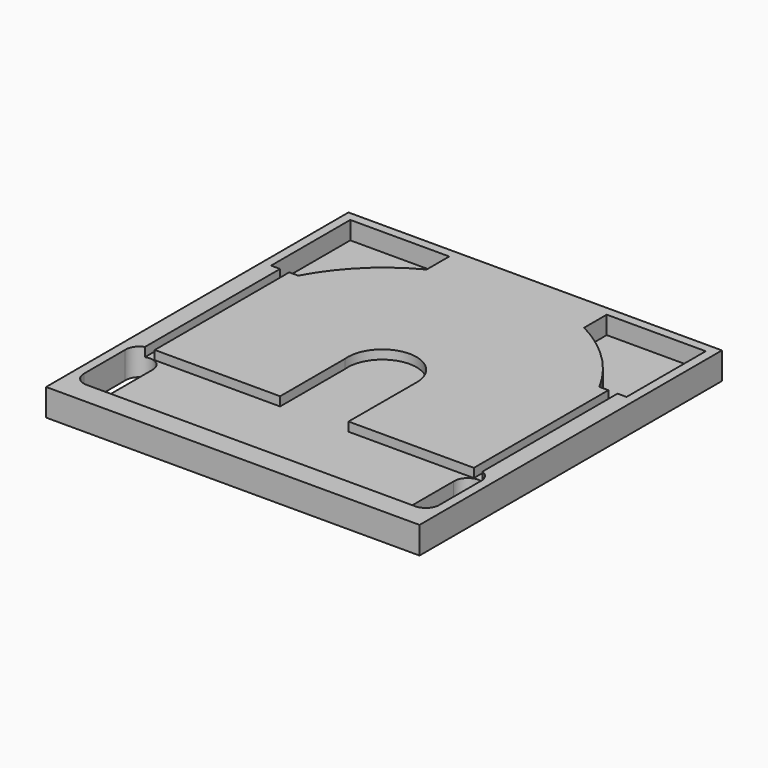
from build123d import *

# Parameters (mm, degrees)
F0_W      = 269.875
F0_H      = 273.05
F1_DEPTH  = 19.05
F3_DEPTH  = 12.7
F5_DEPTH  = 19.05
F6_W      = 3.175
F6_H      = 273.05
F7_DEPTH  = 19.05
F8_W      = 263.525
F8_H      = 3.175
F9_DEPTH  = 19.05
F11_DEPTH = 6.35
F13_DEPTH = 6.35
F14_W     = 263.525
F14_H     = 3.175
F15_DEPTH = 19.05


# Not quite as in the source:
# - ends of sketch curves that miss each other by under 0.0002 mm in the source are joined


with BuildPart() as f1:
    # F0 (on Top) → F1 (new body)
    with BuildSketch(Plane.XY):
        Rectangle(F0_W, F0_H)
    extrude(amount=F1_DEPTH)

    # F2 (on face) → F3 (cut)
    with BuildSketch(Plane.XY.offset(19.05)):
        with BuildLine():
            ThreePointArc((55.5625, 107.0944960946), (84.6752951993, 85.9448479137), (106.2558233698, 57.15))
            Line((106.2558233698, 57.15), (125.4125, 57.15))
            Line((125.4125, 57.15), (125.4125, 127))
            Line((125.4125, 127), (55.5625, 127))
            Line((55.5625, 127), (55.5625, 107.0944960946))
        make_face()
        with BuildLine():
            Line((-125.4125, 57.15), (-106.2558233698, 57.15))
            ThreePointArc((-106.2558233698, 57.15), (-84.6752951993, 85.9448479137), (-55.5625, 107.0944960946))
            Line((-55.5625, 107.0944960946), (-55.5625, 127))
            Line((-55.5625, 127), (-125.4125, 127))
            Line((-125.4125, 127), (-125.4125, 57.15))
        make_face()
    extrude(amount=-F3_DEPTH, mode=Mode.SUBTRACT)

    # F4 (on face) → F5 (cut, through all)
    with BuildSketch(Plane.XY.offset(19.05)):
        with BuildLine():
            Line((-106.3625, -107.9627), (-106.3625, -71.4977328139))
            ThreePointArc((-106.3625, -71.4977328139), (-115.8875, -61.468), (-125.4125, -71.4977328139))
            Line((-125.4125, -71.4977328139), (-125.4125, -107.9627))
            Line((-125.4125, -107.9627), (-125.3998, -107.9627))
            ThreePointArc((-125.3998, -107.9627), (-115.8875, -117.475), (-106.3752, -107.9627))
            Line((-106.3752, -107.9627), (-106.3625, -107.9627))
        make_face()
        with BuildLine():
            ThreePointArc((125.4125, -71.4977328139), (115.8875, -61.468), (106.3625, -71.4977328139))
            Line((106.3625, -71.4977328139), (106.3625, -107.228528768))
            ThreePointArc((106.3625, -107.228528768), (115.8875, -117.475), (125.4125, -107.228528768))
            Line((125.4125, -107.228528768), (125.4125, -71.4977328139))
        make_face()
    extrude(amount=-F5_DEPTH, mode=Mode.SUBTRACT)

    # F6 (on face) → F7 (cut, through all)
    with BuildSketch(Plane.XY.offset(19.05)):
        with Locations((-133.35, 0)):
            Rectangle(F6_W, F6_H)
        with Locations((133.35, 0)):
            Rectangle(F6_W, F6_H)
    extrude(amount=-F7_DEPTH, mode=Mode.SUBTRACT)

    # F8 (on face) → F9 (cut, through all)
    with BuildSketch(Plane.XY.offset(19.05)):
        with Locations((0, 134.9375)):
            Rectangle(F8_W, F8_H)
    extrude(amount=-F9_DEPTH, mode=Mode.SUBTRACT)

    # F10 (on face) → F11 (cut)
    with BuildSketch(Plane.XY.offset(19.05)):
        with BuildLine():
            Line((24.2490875216, -2.6255133905), (24.253090398, -0.6476470458))
            ThreePointArc((24.253090398, -0.6476470458), (-1.7785482929, 22.6185422911), (-24.13, -4.2026132727))
            Line((-24.13, -4.2026132727), (-24.13, -61.468))
            Line((-24.13, -61.468), (-115.8875, -61.468))
            ThreePointArc((-115.8875, -61.468), (-108.9715552829, -64.4377908989), (-106.3625, -71.4977328139))
            Line((-106.3625, -71.4977328139), (-106.3625, -107.9627))
            Line((-106.3625, -107.9627), (-106.3752, -107.9627))
            ThreePointArc((-106.3752, -107.9627), (-109.1568025344, -114.6844232103), (-115.8748084893, -117.4749915334))
            Line((-115.8748084893, -117.4749915334), (115.8875, -117.475))
            ThreePointArc((115.8875, -117.475), (108.892576882, -114.4269988445), (106.3625, -107.228528768))
            Line((106.3625, -107.228528768), (106.3625, -71.4977328139))
            ThreePointArc((106.3625, -71.4977328139), (108.9715552829, -64.4377908989), (115.8875, -61.468))
            Line((115.8875, -61.468), (24.13, -61.468))
            Line((24.13, -61.468), (24.2490875216, -2.6255133905))
        make_face()
    extrude(amount=-F11_DEPTH, mode=Mode.SUBTRACT)

    # F12 (on face) → F13 (cut)
    with BuildSketch(Plane.XY.offset(19.05)):
        with BuildLine():
            Line((119.0726616849, 57.15), (112.5956616849, 57.15))
            Line((112.5956616849, 57.15), (112.5956616849, -61.468))
            Line((112.5956616849, -61.468), (115.8875, -61.468))
            ThreePointArc((115.8875, -61.468), (117.5034429216, -61.6058888442), (119.0726616849, -62.0155683919))
            Line((119.0726616849, -62.0155683919), (119.0726616849, 57.15))
        make_face()
        with BuildLine():
            Line((-115.8341616849, -61.468), (-112.5956616849, -61.468))
            Line((-112.5956616849, -61.468), (-112.5956616849, 57.15))
            Line((-112.5956616849, 57.15), (-119.0726616849, 57.15))
            Line((-119.0726616849, 57.15), (-119.0726616849, -61.468))
            Line((-119.0726616849, -61.468), (-119.0726616849, -62.0155683919))
            ThreePointArc((-119.0726616849, -62.0155683919), (-117.4763944176, -61.6058567373), (-115.8341616849, -61.468))
        make_face()
    extrude(amount=-F13_DEPTH, mode=Mode.SUBTRACT)

    # F14 (on face) → F15 (cut, through all)
    with BuildSketch(Plane.XY.offset(19.05)):
        with Locations((0, -134.9375)):
            Rectangle(F14_W, F14_H)
    extrude(amount=-F15_DEPTH, mode=Mode.SUBTRACT)


solid = f1.part
